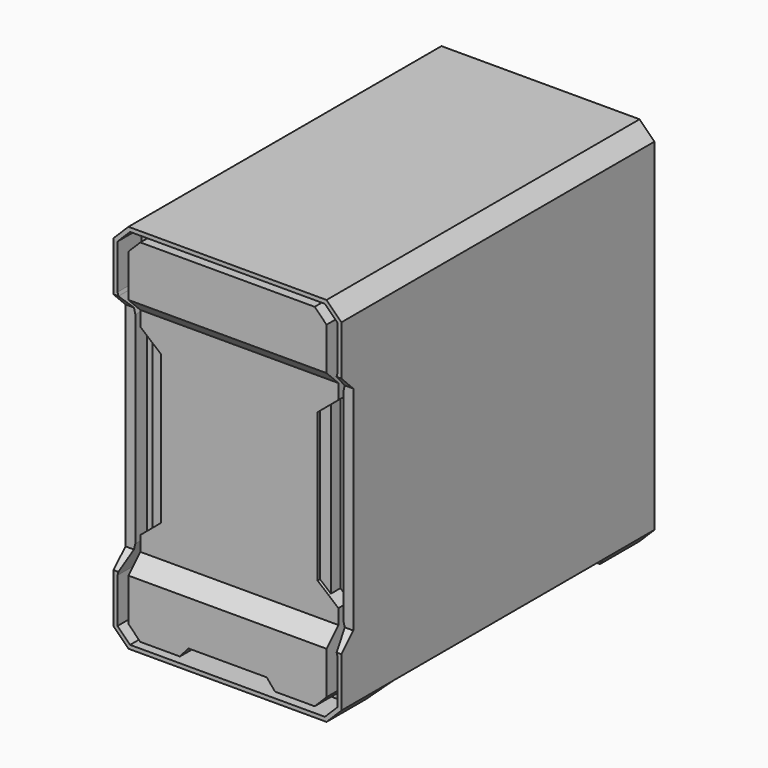
from build123d import *

# Parameters (mm, degrees)
F0_W     = 230
F0_H     = 375
F1_DEPTH = 395
F2_SIZE  = 15
F4_DEPTH = 230.001
F6_DEPTH = 30
F8_DEPTH = 3


with BuildPart() as f1:
    # F0 (on Front) → F1 (new body)
    with BuildSketch(Plane.XZ):
        with Locations((115, 187.5)):
            Rectangle(F0_W, F0_H)
    extrude(amount=-F1_DEPTH)

    # F2
    f2_edges = [f1.edges().sort_by_distance(p)[0] for p in [
        (0, 197.5, 375),
        (0, 197.5, 0),
        (230, 197.5, 375),
        (230, 197.5, 0),
    ]]
    chamfer(f2_edges, length=F2_SIZE)

    # F3 (on face) → F4 (cut, through all)
    with BuildSketch(Plane(origin=(0, 0, 0), x_dir=(0, -1, 0), z_dir=(-1, 0, 0))):
        Polygon((-50, 0), (-65, 15), (-330, 15), (-345, 0), align=None)
        Polygon((-15, 80), (0, 65), (0, 310), (-15, 295), align=None)
    extrude(amount=-F4_DEPTH, mode=Mode.SUBTRACT)

    # F5 (on face) → F6 (cut)
    with BuildSketch(Plane.XZ):
        Polygon((15, 280), (15, 310), (4.8357864376, 310), (10, 289.3431457505), (10, 85.6568542495), (4, 61.6568542495), (4, 16.6568542495), (16.6568542495, 4), (115, 4), (213.3431457505, 4), (226, 16.6568542495), (226, 61.6568542495), (220, 85.6568542495), (220, 289.3431457505), (225.1642135624, 310), (215, 310), (215, 280), (205, 271.6090036882), (205, 103.3909963118), (215, 95), (215, 22), (203, 10), (163, 10), (154.6090036882, 20), (115, 20), (75.3909963118, 20), (67, 10), (27, 10), (15, 22), (15, 95), (25, 103.3909963118), (25, 271.6090036882), align=None)
        Polygon((15, 310), (15, 353), (27, 365), (115, 365), (203, 365), (215, 353), (215, 310), (225.1642135624, 310), (226, 313.3431457505), (226, 358.3431457505), (213.3431457505, 371), (115, 371), (16.6568542495, 371), (4, 358.3431457505), (4, 313.3431457505), (4.8357864376, 310), align=None)
    extrude(amount=-F6_DEPTH, mode=Mode.SUBTRACT)

    # F7 (on face) → F8 (cut)
    with BuildSketch(Plane.XZ.offset(-15)):
        Polygon((36, 262.3789077453), (25, 271.6090036882), (25, 103.3909963118), (36, 112.6210922547), align=None)
        Polygon((205, 103.3909963118), (205, 271.6090036882), (194, 262.3789077453), (194, 112.6210922547), align=None)
    extrude(amount=-F8_DEPTH, mode=Mode.SUBTRACT)


solid = f1.part
